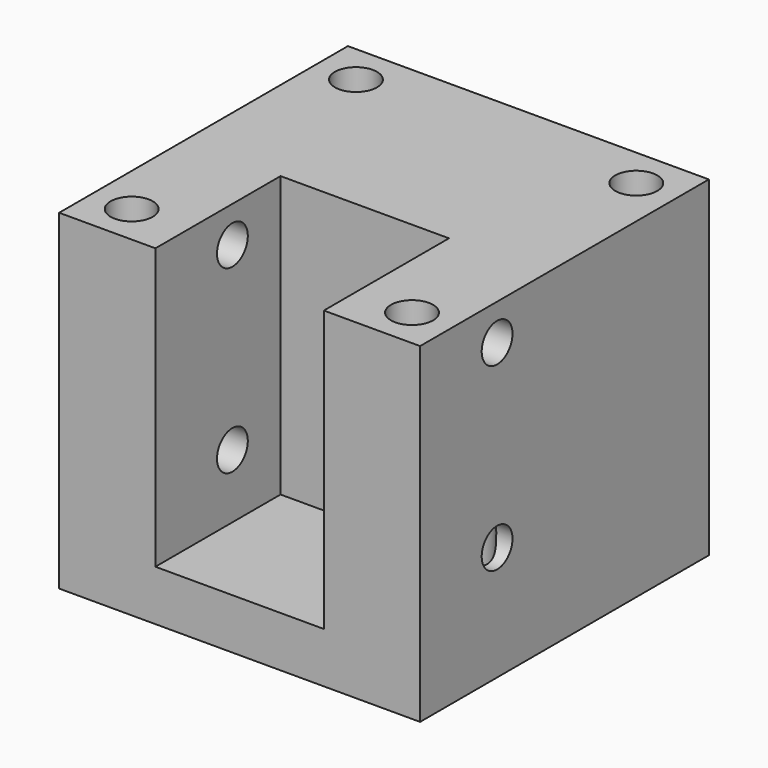
from build123d import *

# Parameters (mm, degrees)
F0_W      = 30
F0_H      = 30
F1_DEPTH  = 27.5
F2_R      = 1.75
F3_DEPTH  = 27.501
F4_R      = 2
F5_DEPTH  = 20
F6_R      = 2
F7_W      = 14
F7_H      = 13
F8_DEPTH  = 23.3
F9_R      = 1.6
F10_DEPTH = 30.001


# Not quite as in the source:
# - a feature names something its author has since deleted; it is built from what else it names


with BuildPart() as f1:
    # F0 (on Top) → F1 (new body)
    with BuildSketch(Plane.XY):
        Rectangle(F0_W, F0_H)
    extrude(amount=F1_DEPTH)

    # F2 (on face) → F3 (cut, through all)
    with BuildSketch(Plane.XY.offset(27.5)):
        with Locations((-11.65, 11.65)):
            Circle(F2_R)
        with Locations((-11.65, -11.65)):
            Circle(F2_R)
        with Locations((11.65, 11.65)):
            Circle(F2_R)
        with Locations((11.65, -11.65)):
            Circle(F2_R)
    extrude(amount=-F3_DEPTH, mode=Mode.SUBTRACT)

    # F4 (on face) → F5 (cut)
    with BuildSketch(Plane(origin=(0, 0, 0), x_dir=(1, 0, 0), z_dir=(0, 0, -1))):
        with Locations((-11.95, 6.6)):
            Circle(F4_R)
        with Locations((12.05, 6.6)):
            Circle(F4_R)
    extrude(amount=-F5_DEPTH, mode=Mode.SUBTRACT)

    # F6
    f6_edges = [f1.edges().sort_by_distance(p)[0] for p in [
        (-13.95, -6.6, 20),
        (10.05, -6.6, 20),
    ]]
    fillet(f6_edges, radius=F6_R)

    # F7 (on face) → F8 (cut)
    with BuildSketch(Plane.XY.offset(27.5)):
        with Locations((0, -8.5)):
            Rectangle(F7_W, F7_H)
    extrude(amount=-F8_DEPTH, mode=Mode.SUBTRACT)

    # F9 (on face) → F10 (cut, through all)
    with BuildSketch(Plane(origin=(-15, 0, 0), x_dir=(0, -1, 0), z_dir=(-1, 0, 0))):
        with Locations((7, 9.5)):
            Circle(F9_R)
        with Locations((7, 24.5)):
            Circle(F9_R)
    extrude(amount=-F10_DEPTH, mode=Mode.SUBTRACT)


solid = f1.part
